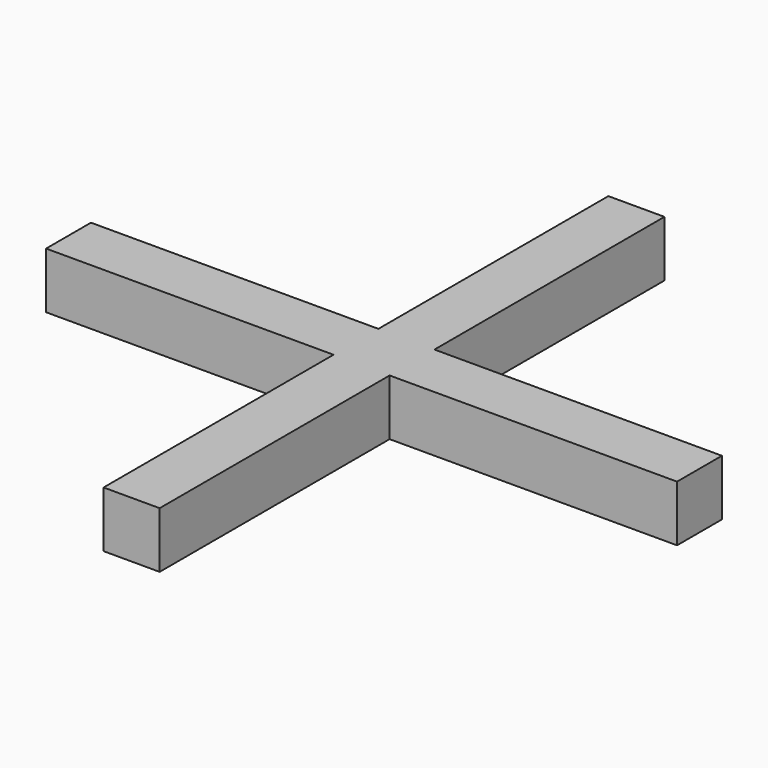
from build123d import *

# Parameters (mm, degrees)
F1_W     = 25.4
F1_H     = 285.75
F2_DEPTH = 25.4
F0_W     = 285.75
F0_H     = 25.4
F3_DEPTH = 25.4


# Not quite as in the source:
# - the program builds the solid bodies; features that only make, move or delete a surface that nothing else refers to are left out


with BuildPart() as f2:
    # F1 (on Top) → F2 (new body)
    with BuildSketch(Plane.XY):
        Rectangle(F1_W, F1_H)
    extrude(amount=F2_DEPTH)

    # F0 (on Top) → F3 (join)
    with BuildSketch(Plane.XY):
        Rectangle(F0_W, F0_H)
    extrude(amount=F3_DEPTH)


solid = f2.part
